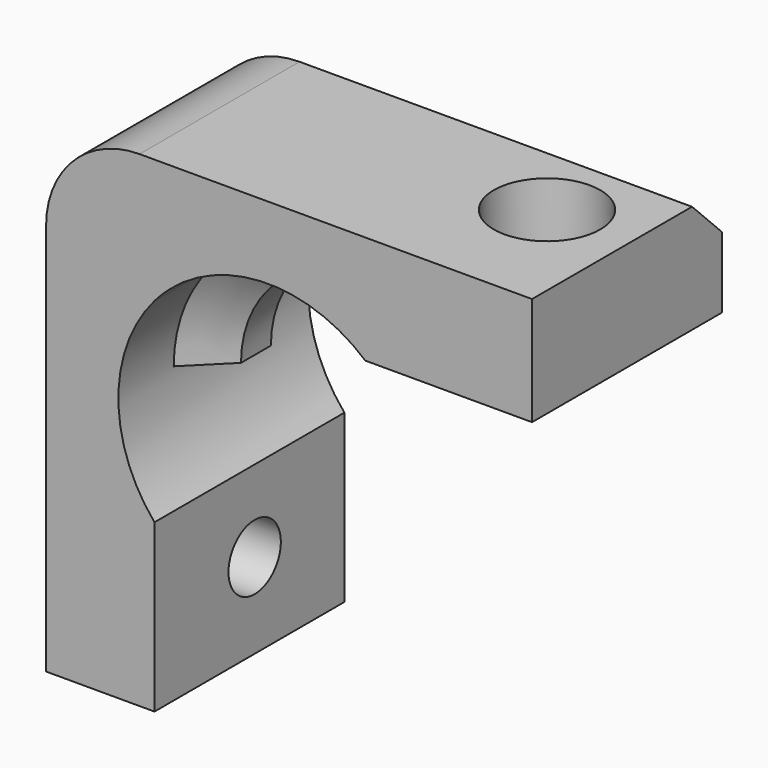
from build123d import *

# Parameters (mm, degrees)
F1_DEPTH     = 12.7
F3_R         = 1.75
F4_DEPTH     = 26.001
F5_R         = 1.75
F6_DEPTH     = 26.001
F8_DEPTH     = 3
F9_T4_ANGLE  = 188.2705145196
F9_S5_R      = 8
F9_T6_DEPTH  = 11
F9_T10_ANGLE = 188.2705145196
F9_S11_R     = 8
F9_T12_DEPTH = 11
F10_R        = 2.85
F10_R_2      = 1.75
F11_DEPTH    = 3
F12_R        = 2.85
F13_DEPTH    = 3
F14_T1_DEPTH = 37.7
F15_SIZE     = 2


# Not quite as in the source:
# - a fillet or chamfer that OpenCascade refuses, or shapes differently, is made with other operations: its cross-section is extruded or revolved along the edge and cut away or added


with BuildPart() as f1:
    # F0 (on Front) → F1 (new body)
    with BuildSketch(Plane.XZ):
        with BuildLine():
            Line((26, 0), (0, 0))
            Line((0, 0), (0, -26))
            Line((0, -26), (5.8, -26))
            Line((5.8, -26), (5.8, -17.0813202825))
            ThreePointArc((5.8, -17.0813202825), (3.8683903961, -11.8683903961), (5.8, -6.6554605098))
            Line((5.8, -6.6554605098), (5.8, -5.8))
            Line((5.8, -5.8), (6.6554605098, -5.8))
            ThreePointArc((6.6554605098, -5.8), (11.8683903961, -3.8683903961), (17.0813202825, -5.8))
            Line((17.0813202825, -5.8), (26, -5.8))
            Line((26, -5.8), (26, 0))
        make_face()
        with BuildLine():
            ThreePointArc((5.8, -6.6554605098), (6.2115361467, -6.2115361467), (6.6554605098, -5.8))
            Line((6.6554605098, -5.8), (5.8, -5.8))
            Line((5.8, -5.8), (5.8, -6.6554605098))
        make_face()
    extrude(amount=F1_DEPTH)

    # F3 (on face) → F4 (cut, through all)
    with BuildSketch(Plane.XY):
        with Locations((21.442, -6)):
            Circle(F3_R)
    extrude(amount=-F4_DEPTH, mode=Mode.SUBTRACT)

    # F5 (on face) → F6 (cut, through all)
    with BuildSketch(Plane(origin=(0, 0, 0), x_dir=(0, -1, 0), z_dir=(-1, 0, 0))):
        with Locations((6, -21.442)):
            Circle(F5_R)
    extrude(amount=-F6_DEPTH, mode=Mode.SUBTRACT)

    # F7 (on offset) → F8 (join, symmetric)
    with BuildSketch(Plane(origin=(0, -6, 0), x_dir=(-1, 0, 0), z_dir=(0, 1, 0))):
        with BuildLine():
            ThreePointArc((-3.8683903961, -11.8683903961), (-6.2115361467, -6.2115361467), (-11.8683903961, -3.8683903961))
            Line((-11.8683903961, -3.8683903961), (-11.8683903961, -5.8683903961))
            ThreePointArc((-11.8683903961, -5.8683903961), (-7.625749709, -7.625749709), (-5.8683903961, -11.8683903961))
            Line((-5.8683903961, -11.8683903961), (-3.8683903961, -11.8683903961))
        make_face()
    extrude(amount=F8_DEPTH, both=True)

    # F9: chamfer of 2 on 2 edges, made by hand


with BuildPart() as f9_tool2:
    # F9_s3 → F9_t4 (revolve)
    with BuildSketch(Plane(origin=(10.953058548, 0, -12.6602903485), x_dir=(0, 1, 0), z_dir=(0.6542755714, 0, -0.7562562242))):
        Polygon((-9, 9.2103462012), (-7, 7.2103462012), (-9, 7.2103462012), align=None)
    revolve(axis=Axis((11.8683903961, -9, -11.8683903961), (0, -1, 0)), revolution_arc=F9_T4_ANGLE)

    # F9_s5 → F9_t6 (intersect, symmetric)
    with BuildSketch(Plane.XZ.offset(8)):
        with Locations((11.8683903961, -11.8683903961)):
            Circle(F9_S5_R)
    extrude(amount=F9_T6_DEPTH, both=True, mode=Mode.INTERSECT)


with BuildPart() as f1_1:
    add(f1.part)

    # F9_t1: cut F9_tool2
    add(f9_tool2.part, mode=Mode.SUBTRACT)


with BuildPart() as f9_tool8:
    # F9_s9 → F9_t10 (revolve)
    with BuildSketch(Plane(origin=(10.953058548, 0, -12.6602903485), x_dir=(0, 1, 0), z_dir=(0.6542755714, 0, -0.7562562242))):
        Polygon((-3, 9.2103462012), (-5, 7.2103462012), (-3, 7.2103462012), align=None)
    revolve(axis=Axis((11.8683903961, -3, -11.8683903961), (0, -1, 0)), revolution_arc=F9_T10_ANGLE)

    # F9_s11 → F9_t12 (intersect, symmetric)
    with BuildSketch(Plane.XZ.offset(4)):
        with Locations((11.8683903961, -11.8683903961)):
            Circle(F9_S11_R)
    extrude(amount=F9_T12_DEPTH, both=True, mode=Mode.INTERSECT)


with BuildPart() as f1_2:
    add(f1_1.part)

    # F9_t7: cut F9_tool8
    add(f9_tool8.part, mode=Mode.SUBTRACT)

    # F10 (on face) → F11 (cut)
    with BuildSketch(Plane(origin=(0, 0, 0), x_dir=(0, -1, 0), z_dir=(-1, 0, 0))):
        with Locations((6, -21.442)):
            Circle(F10_R)
        with Locations((6, -21.442)):
            Circle(F10_R_2, mode=Mode.SUBTRACT)
    extrude(amount=-F11_DEPTH, mode=Mode.SUBTRACT)

    # F12 (on face) → F13 (cut)
    with BuildSketch(Plane.XY):
        with Locations((21.442, -6)):
            Circle(F12_R)
    extrude(amount=-F13_DEPTH, mode=Mode.SUBTRACT)

    # F14: fillet of radius 5 on 1 edges, made by hand

    # F14_s2 → F14_t1 (cut)
    with BuildSketch(Plane.XZ.offset(-12.5)):
        with BuildLine():
            ThreePointArc((5, 0), (1.4644660941, -1.4644660941), (0, -5))
            Line((0, -5), (0, 0))
            Line((0, 0), (5, 0))
        make_face()
    extrude(amount=F14_T1_DEPTH, mode=Mode.SUBTRACT)

    # F15
    f15_edges = [f1_2.edges().sort_by_distance(p)[0] for p in [
        (0, 0, -15.5),
        (1.464466, 0, -1.464466),
        (15.5, 0, 0),
    ]]
    chamfer(f15_edges, length=F15_SIZE)


solid = f1_2.part
